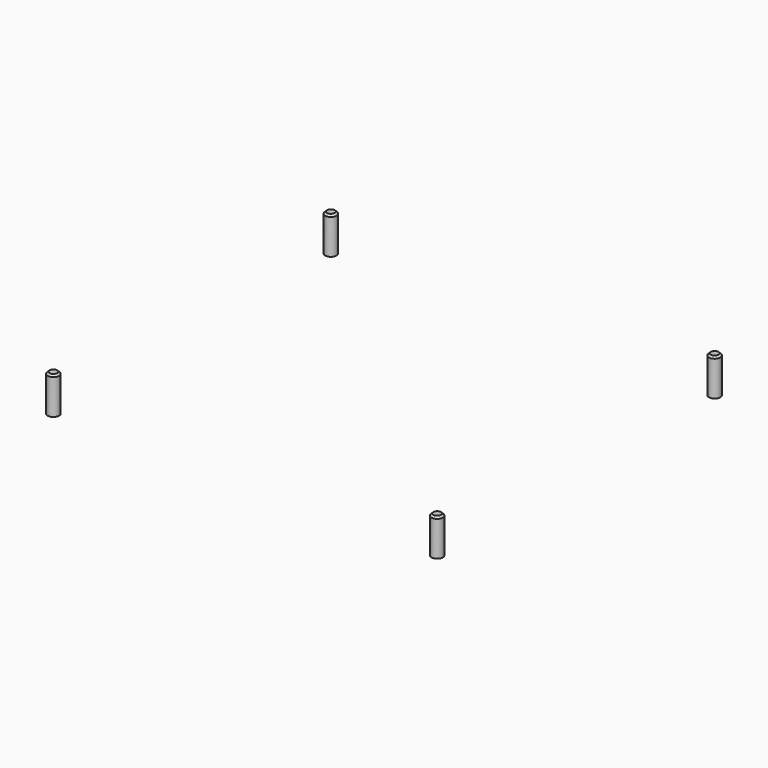
from build123d import *

# Parameters (mm, degrees)
F0_R      = 1.55
F5_DEPTH  = 5
F6_SIZE   = 0.5
F7_DEPTH  = 5
F8_SIZE   = 0.5
F9_DEPTH  = 5
F10_SIZE  = 0.5
F11_DEPTH = 5
F12_SIZE  = 0.5


# Not quite as in the source:
# - the program builds the solid bodies; features that only make, move or delete a surface that nothing else refers to are left out


with BuildPart() as f5:
    # F0 (on Top) → F5 (new body, symmetric)
    with BuildSketch(Plane.XY):
        with Locations((-62.5403363705, -52.2236271612)):
            Circle(F0_R)
    extrude(amount=F5_DEPTH, both=True)

    # F6
    f6_edges = [f5.edges().sort_by_distance(p)[0] for p in [
        (-64.090336, -52.223627, 5),
    ]]
    chamfer(f6_edges, length=F6_SIZE)


with BuildPart() as f7:
    # F0 (on Top) → F7 (new body, symmetric)
    with BuildSketch(Plane.XY):
        with Locations((41.4596636295, -52.2236271612)):
            Circle(F0_R)
    extrude(amount=F7_DEPTH, both=True)

    # F8
    f8_edges = [f7.edges().sort_by_distance(p)[0] for p in [
        (39.909664, -52.223627, 5),
    ]]
    chamfer(f8_edges, length=F8_SIZE)


with BuildPart() as f9:
    # F0 (on Top) → F9 (new body, symmetric)
    with BuildSketch(Plane.XY):
        with Locations((41.4596636295, 41.7763728388)):
            Circle(F0_R)
    extrude(amount=F9_DEPTH, both=True)

    # F10
    f10_edges = [f9.edges().sort_by_distance(p)[0] for p in [
        (39.909664, 41.776373, 5),
    ]]
    chamfer(f10_edges, length=F10_SIZE)


with BuildPart() as f11:
    # F0 (on Top) → F11 (new body, symmetric)
    with BuildSketch(Plane.XY):
        with Locations((-62.5403363705, 41.7763728388)):
            Circle(F0_R)
    extrude(amount=F11_DEPTH, both=True)

    # F12
    f12_edges = [f11.edges().sort_by_distance(p)[0] for p in [
        (-64.090336, 41.776373, 5),
    ]]
    chamfer(f12_edges, length=F12_SIZE)


solid = Compound([f5.part, f7.part, f9.part, f11.part])
